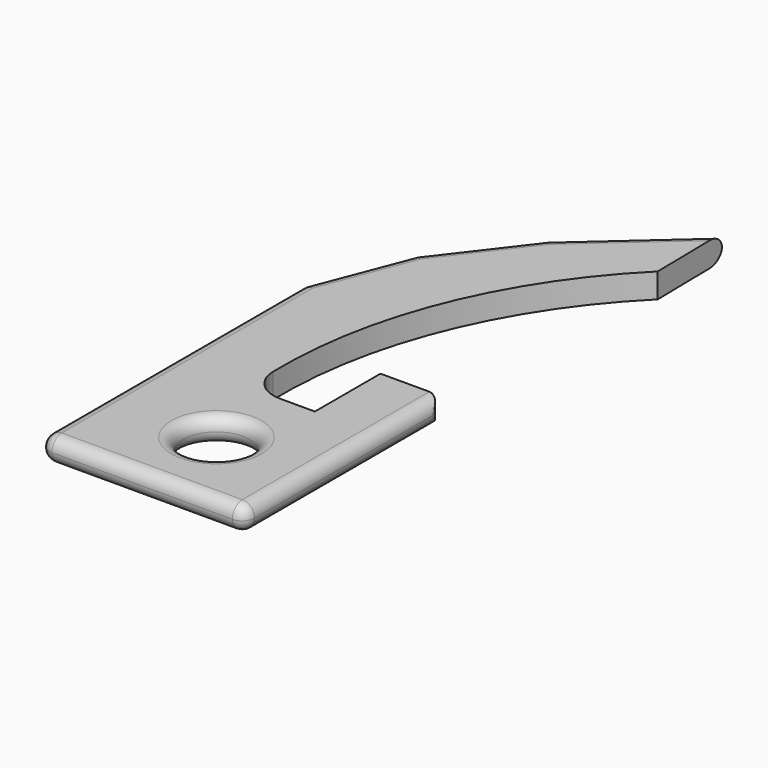
from build123d import *

# Parameters (mm, degrees)
F0_R     = 5.08
F1_DEPTH = 3.81
F2_R     = 1.90499
F4_R     = 5.08


# Not quite as in the source:
# - two fillets or chamfers of one size are made in one step
# - a fillet or chamfer is up to 0.001 mm smaller than in the source, because OpenCascade refuses the exact size


with BuildPart() as f1:
    # F0 (on Top) → F1 (new body)
    with BuildSketch(Plane.XY):
        with BuildLine():
            Line((-5.6879511814, 25.4), (-5.6879511814, -25.4))
            Line((-5.6879511814, -25.4), (5.6879511814, -25.4))
            Line((5.6879511814, -25.4), (26.0620488186, -25.4))
            Line((26.0620488186, -25.4), (26.0620488186, 0))
            Line((26.0620488186, 0), (26.0620488186, 12.7))
            Line((26.0620488186, 12.7), (16.6040229345, 12.7))
            Line((16.6040229345, 12.7), (16.6040229345, 0))
            Line((16.6040229345, 0), (6.4440229345, 0))
            ThreePointArc((6.4440229345, 0), (10.1083489192, 29.4811569654), (26.0620488186, 54.5419901609))
            Line((26.0620488186, 54.5419901609), (25.8431795214, 67.2401040457))
            Line((25.8431795214, 67.2401040457), (10.0171072409, 53.1962551177))
            Line((10.0171072409, 53.1962551177), (0, 40.1331372559))
            Line((0, 40.1331372559), (-5.6879511814, 25.4))
        make_face()
        with Locations((11.5240229345, -12.7)):
            Circle(F0_R, mode=Mode.SUBTRACT)
    extrude(amount=F1_DEPTH)

    # F2 (radius 1.905 in the source; OpenCascade refuses exactly that, so slightly less here)
    f2_edges = [f1.edges().sort_by_distance(p)[0] for p in [
        (-5.687951, 0, 3.81),
        (10.187049, -25.4, 3.81),
        (10.187049, -25.4, 0),
        (26.062049, -6.35, 3.81),
        (26.062049, -6.35, 0),
        (26.062049, -25.4, 1.905),
        (-5.687951, -25.4, 1.905),
        (26.062049, 12.7, 1.905),
        (-2.843976, 32.766569, 3.81),
        (-2.843976, 32.766569, 0),
        (-5.687951, 0, 0),
        (6.444023, -12.7, 0),
        (6.444023, -12.7, 3.81),
        (17.930143, 60.21818, 0),
        (17.930143, 60.21818, 3.81),
        (5.008554, 46.664696, 3.81),
        (-5.687951, 25.4, 1.905),
        (0, 40.133137, 1.905),
        (5.008554, 46.664696, 0),
    ]]
    fillet(f2_edges, radius=F2_R)

    # F4
    f4_edges = [f1.edges().sort_by_distance(p)[0] for p in [
        (6.444023, 0, 1.905),
    ]]
    fillet(f4_edges, radius=F4_R)


solid = f1.part
